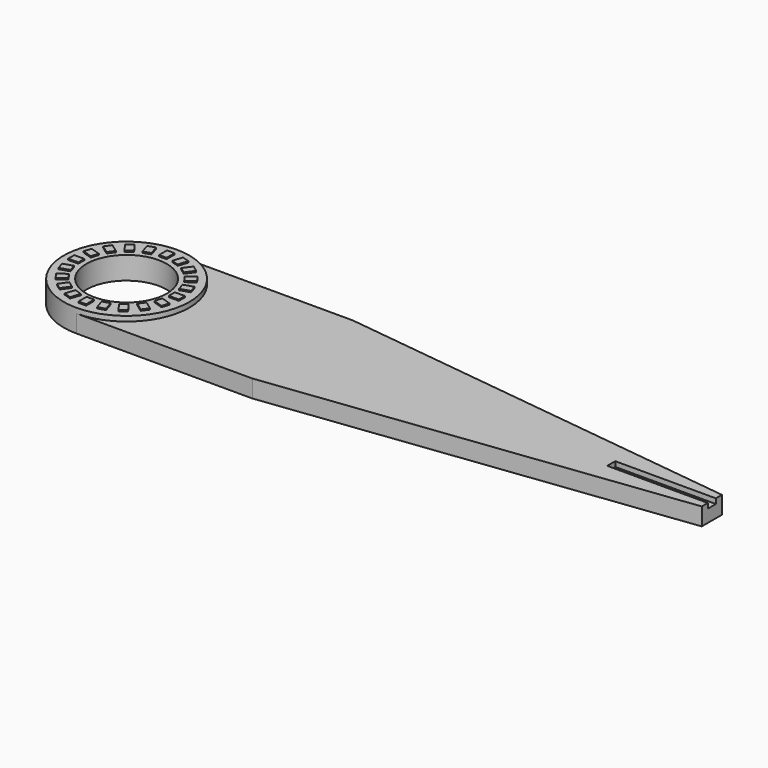
from build123d import *

# Parameters (mm, degrees)
F0_R         = 8
F1_DEPTH     = 3.5
F2_R         = 12.5
F2_R_2       = 8
F3_DEPTH     = 1
F4_W         = 1.5
F4_H         = 2
F4_W_2       = 2
F4_H_2       = 1.5
F5_DEPTH     = 0.25
F6_W         = 20
F6_H         = 2
F7_DEPTH     = 1
F8_TEXT_SIZE = 19.0939288586
F9_DEPTH     = 1


# Not quite as in the source:
# - Text() gives the source's letters only with a copy of the font that has no kerning and outlines rounded to 1/6400 em; it was checked with that copy


with BuildPart() as f1:
    # F0 (on Top) → F1 (new body)
    with BuildSketch(Plane.XY):
        with BuildLine():
            ThreePointArc((0, -12.5), (8.8388347648, -8.8388347648), (12.5, 0))
            ThreePointArc((12.5, 0), (8.8388347648, 8.8388347648), (0, 12.5))
            ThreePointArc((0, 12.5), (-12.5, 0), (0, -12.5))
        make_face()
        Circle(F0_R, mode=Mode.SUBTRACT)
        with BuildLine():
            ThreePointArc((0, 12.5), (8.8388347648, 8.8388347648), (12.5, 0))
            ThreePointArc((12.5, 0), (8.8388347648, -8.8388347648), (0, -12.5))
            Line((0, -12.5), (35, -12.5))
            Line((35, -12.5), (116.3887844346, -2.5067138408))
            Line((116.3887844346, -2.5067138408), (116.3887844346, 2.5067138408))
            Line((116.3887844346, 2.5067138408), (35, 12.5))
            Line((35, 12.5), (0, 12.5))
        make_face()
    extrude(amount=F1_DEPTH)

    # F2 (on face) → F3 (join)
    with BuildSketch(Plane.XY.offset(3.5)):
        Circle(F2_R)
        Circle(F2_R_2, mode=Mode.SUBTRACT)
    extrude(amount=F3_DEPTH)

    # F4 (on face) → F5 (join)
    with BuildSketch(Plane.XY.offset(4.5)):
        with Locations((0, 10)):
            Rectangle(F4_W, F4_H)
        Polygon((-2.6858945509, 10.693384425), (-4.1124793253, 10.2298589335), (-3.4944453366, 8.3277459009), (-2.0678605622, 8.7912713924), align=None)
        Polygon((-5.8588750294, 9.3400258773), (-7.072400521, 8.4583479989), (-5.8968300164, 6.8403140102), (-4.6833045249, 7.7219918886), align=None)
        Polygon((-8.4583479989, 7.072400521), (-9.3400258773, 5.8588750294), (-7.7219918886, 4.6833045249), (-6.8403140102, 5.8968300164), align=None)
        Polygon((-10.2298589335, 4.1124793253), (-10.693384425, 2.6858945509), (-8.7912713924, 2.0678605622), (-8.3277459009, 3.4944453366), align=None)
        with Locations((-10, 0)):
            Rectangle(F4_W_2, F4_H_2)
        Polygon((-10.693384425, -2.6858945509), (-10.2298589335, -4.1124793253), (-8.3277459009, -3.4944453366), (-8.7912713924, -2.0678605622), align=None)
        Polygon((-9.3400258773, -5.8588750294), (-8.4583479989, -7.072400521), (-6.8403140102, -5.8968300164), (-7.7219918886, -4.6833045249), align=None)
        Polygon((-7.072400521, -8.4583479989), (-5.8588750294, -9.3400258773), (-4.6833045249, -7.7219918886), (-5.8968300164, -6.8403140102), align=None)
        Polygon((-4.1124793253, -10.2298589335), (-2.6858945509, -10.693384425), (-2.0678605622, -8.7912713924), (-3.4944453366, -8.3277459009), align=None)
        with Locations((0, -10)):
            Rectangle(F4_W, F4_H)
        Polygon((2.6858945509, -10.693384425), (4.1124793253, -10.2298589335), (3.4944453366, -8.3277459009), (2.0678605622, -8.7912713924), align=None)
        Polygon((5.8588750294, -9.3400258773), (7.072400521, -8.4583479989), (5.8968300164, -6.8403140102), (4.6833045249, -7.7219918886), align=None)
        Polygon((8.4583479989, -7.072400521), (9.3400258773, -5.8588750294), (7.7219918886, -4.6833045249), (6.8403140102, -5.8968300164), align=None)
        Polygon((10.2298589335, -4.1124793253), (10.693384425, -2.6858945509), (8.7912713924, -2.0678605622), (8.3277459009, -3.4944453366), align=None)
        with Locations((10, 0)):
            Rectangle(F4_W_2, F4_H_2)
        Polygon((10.693384425, 2.6858945509), (10.2298589335, 4.1124793253), (8.3277459009, 3.4944453366), (8.7912713924, 2.0678605622), align=None)
        Polygon((9.3400258773, 5.8588750294), (8.4583479989, 7.072400521), (6.8403140102, 5.8968300164), (7.7219918886, 4.6833045249), align=None)
        Polygon((7.072400521, 8.4583479989), (5.8588750294, 9.3400258773), (4.6833045249, 7.7219918886), (5.8968300164, 6.8403140102), align=None)
        Polygon((4.1124793253, 10.2298589335), (2.6858945509, 10.693384425), (2.0678605622, 8.7912713924), (3.4944453366, 8.3277459009), align=None)
    extrude(amount=F5_DEPTH)

    # F6 (on face) → F7 (cut)
    with BuildSketch(Plane.XY.offset(3.5)):
        with Locations((106.3887844346, -0.0067138408)):
            Rectangle(F6_W, F6_H)
    extrude(amount=-F7_DEPTH, mode=Mode.SUBTRACT)

    # F8 (on face) → F9 (join)
    with BuildSketch(Plane(origin=(0, 0, 0), x_dir=(1, 0, 0), z_dir=(0, 0, -1))):
        with Locations((13.521714136, -7.0232450962)):
            Text('K.I-T', F8_TEXT_SIZE, font='Arimo', font_style=FontStyle.ITALIC, text_align=(TextAlign.LEFT, TextAlign.BOTTOM))
    extrude(amount=F9_DEPTH)


solid = f1.part
